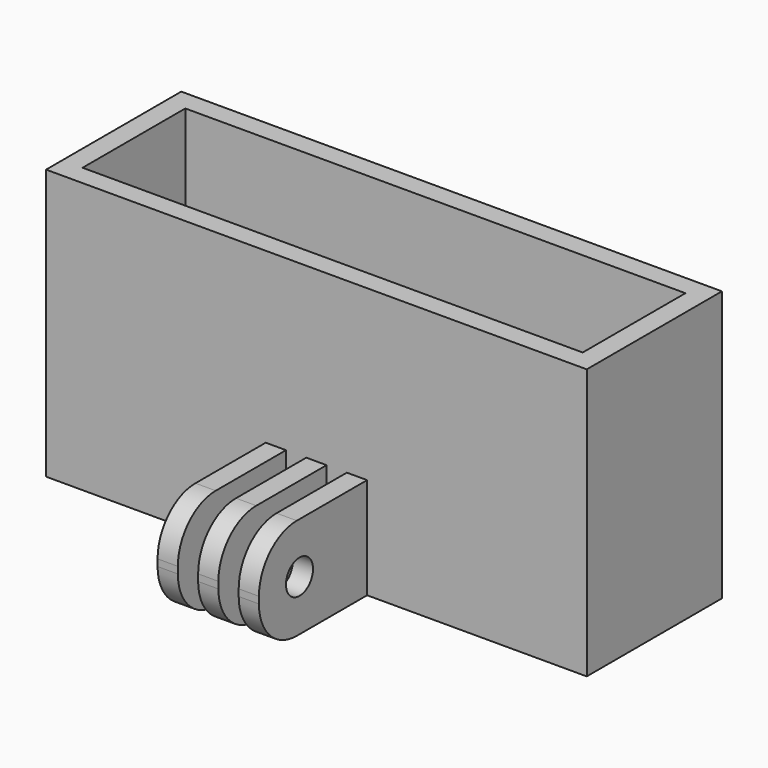
from build123d import *

# Parameters (mm, degrees)
F0_W          = 80
F0_H          = 25
F1_DEPTH      = 40
F2_W          = 3
F2_H          = 20
F3_DEPTH      = 15
F4_R          = 7
F5_R          = 7
F7_D          = 5
F9_D          = 5
F10_T         = 3
F10_T3_DEPTH  = 21
F10_T5_DEPTH  = 9
F10_T7_DEPTH  = 9
F10_T9_DEPTH  = 9
F10_T11_DEPTH = 9
F10_T13_DEPTH = 9


# Not quite as in the source:
# - a shell that OpenCascade refuses in one call is made with other operations: the cavity is built on its own and cut out


with BuildPart() as f1:
    # F0 (on Top) → F1 (new body)
    with BuildSketch(Plane.XY):
        Rectangle(F0_W, F0_H)
    extrude(amount=F1_DEPTH)

    # F2 (on face) → F3 (join)
    with BuildSketch(Plane(origin=(0, 0, 0), x_dir=(1, 0, 0), z_dir=(0, 0, -1))):
        with Locations((-6, 22.5)):
            Rectangle(F2_W, F2_H)
        with Locations((0, 22.5)):
            Rectangle(F2_W, F2_H)
        with Locations((6, 22.5)):
            Rectangle(F2_W, F2_H)
        with Locations((3, -22.5)):
            Rectangle(F2_W, F2_H)
        with Locations((-3, -22.5)):
            Rectangle(F2_W, F2_H)
    extrude(amount=-F3_DEPTH)

    # F4
    f4_edges = [f1.edges().sort_by_distance(p)[0] for p in [
        (3, 32.5, 0),
        (-3, 32.5, 0),
        (-3, 32.5, 15),
        (3, 32.5, 15),
    ]]
    fillet(f4_edges, radius=F4_R)

    # F5
    f5_edges = [f1.edges().sort_by_distance(p)[0] for p in [
        (-6, -32.5, 15),
        (0, -32.5, 15),
        (6, -32.5, 15),
        (6, -32.5, 0),
        (0, -32.5, 0),
        (-6, -32.5, 0),
    ]]
    fillet(f5_edges, radius=F5_R)

    # F7 (through all)
    with Locations(Plane(origin=(-7.5, 0, 0), x_dir=(0, -1, 0), z_dir=(-1, 0, 0))):
        with Locations((25, 7.5)):
            Hole(F7_D / 2)

    # F9 (through all)
    with Locations(Plane(origin=(-4.5, 0, 0), x_dir=(0, -1, 0), z_dir=(-1, 0, 0))):
        with Locations((-23.3794022352, 7.5034750625)):
            Hole(F9_D / 2)

    # F10: shell of thickness 3, made by hand


with BuildPart() as f10_core1:
    # F10_t2: copy of F1
    add(f1.part)

    # the walls: a layer under each face that stays
    f10_faces = [f10_core1.faces().sort_by_distance(p)[0] for p in [
        (0, 0, 0),
        (7.5, -15.8333333333, 12.5),
        (6, -30.4497474683, 2.0502525317),
        (0, -12.5, 20),
        (4.5, -29.1666666667, 12.5),
        (40, 0, 20),
        (0, 12.5, 20),
        (1.5, -15.8333333333, 12.5),
        (4.5, 29.1666666667, 12.5),
        (0, -30.4497474683, 2.0502525317),
        (3, 30.4497474683, 2.0502525317),
        (-1.5, -29.1666666667, 12.5),
        (1.5, 15.8333333333, 12.5),
        (-4.5, -15.8333333333, 12.5),
        (-1.5, 29.1666666667, 12.5),
        (-6, -30.4497474683, 2.0502525317),
        (-3, 30.4497474683, 2.0502525317),
        (-7.5, -29.1666666667, 12.5),
        (-4.5, 15.8333333333, 12.5),
        (-40, 0, 20),
        (6, -32.5, 7.5),
        (6, -30.4497474683, 12.9497474683),
        (6, -19, 15),
        (6, -22.5, 7.5),
        (-6, -19, 15),
        (0, -19, 15),
        (3, 19, 15),
        (-3, 19, 15),
        (0, -32.5, 7.5),
        (0, -30.4497474683, 12.9497474683),
        (0, -22.5, 7.5),
        (3, 32.5, 7.5),
        (3, 30.4497474683, 12.9497474683),
        (3, 25.8794022352, 7.5034750625),
        (-6, -32.5, 7.5),
        (-6, -30.4497474683, 12.9497474683),
        (-6, -22.5, 7.5),
        (-3, 32.5, 7.5),
        (-3, 30.4497474683, 12.9497474683),
        (-3, 25.8794022352, 7.5034750625),
    ]]
    thicken(f10_faces, amount=-F10_T, mode=Mode.SUBTRACT)

    # F10_s4 → F10_t3 (cut)
    with BuildSketch(Plane.XY.offset(-3)):
        Polygon((7.53, -12.53), (4.5, -12.5), (4.5, -9.5), (7.5, -9.5), align=None)
        Polygon((-7.53, -12.53), (-7.5, -9.5), (-4.5, -9.5), (-4.5, -12.5), align=None)
        Polygon((-4.47, -12.53), (-4.5, -9.5), (-7.5, -9.5), (-7.5, -12.5), align=None)
        Polygon((-1.53, -12.53), (-1.5, -9.5), (1.5, -9.5), (1.5, -12.5), align=None)
        Polygon((1.53, -12.53), (1.5, -9.5), (-1.5, -9.5), (-1.5, -12.5), align=None)
        Polygon((4.47, -12.53), (4.5, -9.5), (7.5, -9.5), (7.5, -12.5), align=None)
        Polygon((4.53, 12.53), (4.5, 9.5), (1.5, 9.5), (1.5, 12.5), align=None)
        Polygon((1.47, 12.53), (1.5, 9.5), (4.5, 9.5), (4.5, 12.5), align=None)
        Polygon((-1.47, 12.53), (-1.5, 9.5), (-4.5, 9.5), (-4.5, 12.5), align=None)
        Polygon((-4.53, 12.53), (-4.5, 9.5), (-1.5, 9.5), (-1.5, 12.5), align=None)
    extrude(amount=F10_T3_DEPTH, mode=Mode.SUBTRACT)

    # F10_s6 → F10_t5 (cut)
    with BuildSketch(Plane.YZ.offset(-10.5)):
        Polygon((-12.53, 15.03), (-9.5, 15), (-9.5, 12), (-12.5, 12), align=None)
    extrude(amount=F10_T5_DEPTH, mode=Mode.SUBTRACT)

    # F10_s8 → F10_t7 (cut)
    with BuildSketch(Plane.YZ.offset(-4.5)):
        Polygon((-12.53, 15.03), (-9.5, 15), (-9.5, 12), (-12.5, 12), align=None)
    extrude(amount=F10_T7_DEPTH, mode=Mode.SUBTRACT)

    # F10_s10 → F10_t9 (cut)
    with BuildSketch(Plane.YZ.offset(1.5)):
        Polygon((-12.53, 15.03), (-9.5, 15), (-9.5, 12), (-12.5, 12), align=None)
    extrude(amount=F10_T9_DEPTH, mode=Mode.SUBTRACT)

    # F10_s12 → F10_t11 (cut)
    with BuildSketch(Plane.YZ.offset(-1.5)):
        Polygon((12.53, 15.03), (9.5, 15), (9.5, 12), (12.5, 12), align=None)
    extrude(amount=F10_T11_DEPTH, mode=Mode.SUBTRACT)

    # F10_s14 → F10_t13 (cut)
    with BuildSketch(Plane.YZ.offset(-7.5)):
        Polygon((12.53, 15.03), (9.5, 15), (9.5, 12), (12.5, 12), align=None)
    extrude(amount=F10_T13_DEPTH, mode=Mode.SUBTRACT)


with BuildPart() as f1_1:
    add(f1.part)

    # what is left inside the walls is the cavity
    f10_cavity = [f10_core1.part.solids().sort_by_distance(p)[0] for p in [
        (0, 9.47, 27.666667),
    ]]
    add(f10_cavity, mode=Mode.SUBTRACT)


solid = f1_1.part
